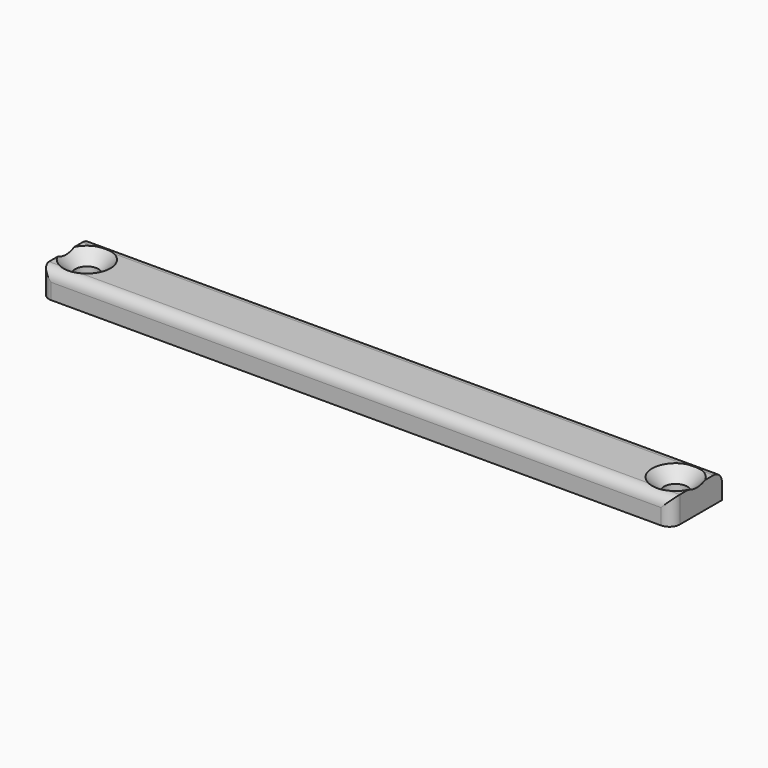
from build123d import *

# Parameters (mm, degrees)
F0_W           = 120
F0_H           = 12
F1_DEPTH       = 5
F3_D           = 4.4
F3_DEPTH       = 18
F3_CSINK_D     = 8.96
F3_CSINK_ANGLE = 90
F3_TIP         = 1.3218933619
F4_T1_DEPTH    = 130
F4_T3_DEPTH    = 15


# Not quite as in the source:
# - a fillet or chamfer that OpenCascade refuses, or shapes differently, is made with other operations: its cross-section is extruded or revolved along the edge and cut away or added


with BuildPart() as f1:
    # F0 (on Top) → F1 (new body)
    with BuildSketch(Plane.XY):
        with Locations((60, 6)):
            Rectangle(F0_W, F0_H)
    extrude(amount=F1_DEPTH)

    # F3
    with Locations(Plane.XY.offset(5)):
        with Locations((4, 6), (116, 6)):
            CounterSinkHole(F3_D / 2, F3_CSINK_D / 2, depth=F3_DEPTH, counter_sink_angle=F3_CSINK_ANGLE)
            with Locations((0, 0, -(F3_DEPTH + F3_TIP / 2))):  # 118° drill point
                Cone(0, F3_D / 2, F3_TIP, mode=Mode.SUBTRACT)

    # F4: fillet of radius 2 on 4 edges, made by hand

    # F4_s2 → F4_t1 (cut)
    with BuildSketch(Plane.YZ.offset(-5)):
        with BuildLine():
            ThreePointArc((0, 3), (0.5857864376, 4.4142135624), (2, 5))
            Line((2, 5), (0, 5))
            Line((0, 5), (0, 3))
        make_face()
        with BuildLine():
            ThreePointArc((10, 5), (11.4142135624, 4.4142135624), (12, 3))
            Line((12, 3), (12, 5))
            Line((12, 5), (10, 5))
        make_face()
    extrude(amount=F4_T1_DEPTH, mode=Mode.SUBTRACT)

    # F4_s4 → F4_t3 (cut)
    with BuildSketch(Plane.XY.offset(-5)):
        with BuildLine():
            ThreePointArc((0, 2), (0.5857864376, 0.5857864376), (2, 0))
            Line((2, 0), (0, 0))
            Line((0, 0), (0, 2))
        make_face()
        with BuildLine():
            ThreePointArc((118, 0), (119.4142135624, 0.5857864376), (120, 2))
            Line((120, 2), (120, 0))
            Line((120, 0), (118, 0))
        make_face()
    extrude(amount=F4_T3_DEPTH, mode=Mode.SUBTRACT)


solid = f1.part
